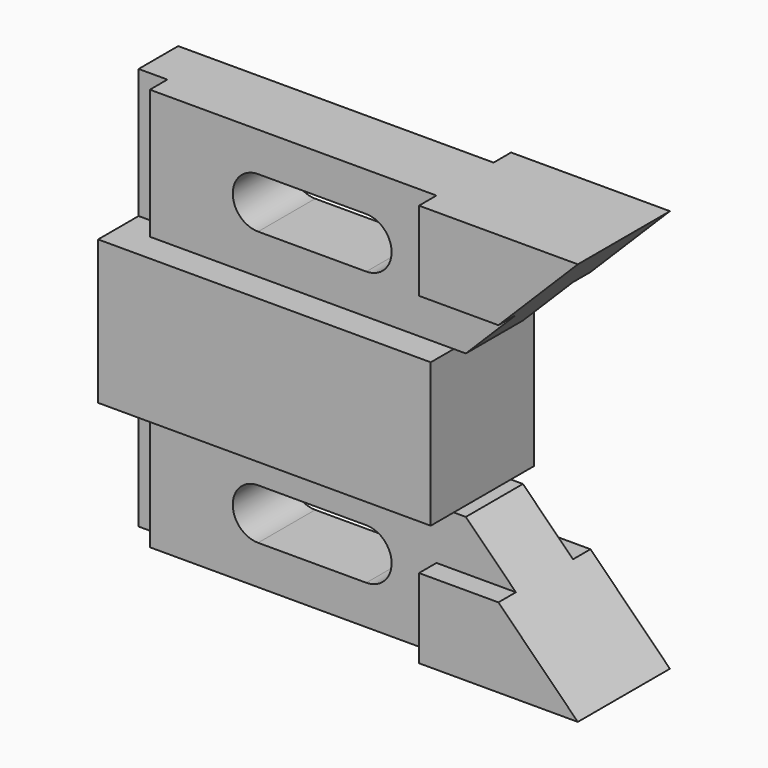
from build123d import *

# Parameters (mm, degrees)
F0_W     = 28.448
F0_H     = 31.75
F1_DEPTH = 73.406
F3_DEPTH = 7.874
F4_W     = 6.35
F4_H     = 28.575
F5_DEPTH = 4.826
F7_DEPTH = 12.7


# Not quite as in the source:
# - a pattern or mirror of a feature is missing from the dataset's text; its kind, count and spacing are read off the source's solid
# - a feature names something its author has since deleted; it is built from what else it names


with BuildPart() as f1:
    # F0 (on Right) → F1 (new body)
    with BuildSketch(Plane.YZ):
        Rectangle(F0_W, F0_H)
    extrude(amount=F1_DEPTH)

    # F2 (on Front) → F3 (join, symmetric)
    with BuildSketch(Plane.XZ):
        Polygon((0, 44.45), (0, 15.875), (73.406, 15.875), (76.073, 15.875), (104.648, 44.45), align=None)
        with BuildLine():
            ThreePointArc((30.226, 24.638), (24.638, 30.226), (30.226, 35.814))
            Line((30.226, 35.814), (54.102, 35.814))
            ThreePointArc((54.102, 35.814), (58.0533126933, 34.1773126933), (59.69, 30.226))
            ThreePointArc((59.69, 30.226), (58.0533126933, 26.2746873067), (54.102, 24.638))
            Line((54.102, 24.638), (30.226, 24.638))
        make_face(mode=Mode.SUBTRACT)
        Polygon((104.648, -44.45), (76.073, -15.875), (73.406, -15.875), (0, -15.875), (0, -44.45), align=None)
        with BuildLine():
            ThreePointArc((54.102, -24.638), (58.0533126933, -26.2746873067), (59.69, -30.226))
            ThreePointArc((59.69, -30.226), (58.0533126933, -34.1773126933), (54.102, -35.814))
            Line((54.102, -35.814), (30.226, -35.814))
            ThreePointArc((30.226, -35.814), (24.638, -30.226), (30.226, -24.638))
            Line((30.226, -24.638), (54.102, -24.638))
        make_face(mode=Mode.SUBTRACT)
    extrude(amount=F3_DEPTH, both=True)

    # F4 (on face) → F5 (cut)
    with BuildSketch(Plane.XZ.offset(7.874)):
        with Locations((3.175, 30.1625)):
            Rectangle(F4_W, F4_H)
    f5 = extrude(amount=-F5_DEPTH, mode=Mode.SUBTRACT)

    # F5_copies: F5 across plane
    add(f5.mirror(Plane(origin=(0, 0, 0), x_dir=(-1, 0, 0), z_dir=(0, 0, -1))), mode=Mode.SUBTRACT)

    # F6 (on Front) → F7 (join, symmetric)
    with BuildSketch(Plane.XZ):
        Polygon((104.648, 44.45), (69.596, 44.45), (69.596, 26.924), (87.122, 26.924), align=None)
    f7 = extrude(amount=F7_DEPTH, both=True)

    # F7_copies: F7 across plane
    add(f7.mirror(Plane(origin=(0, 0, 0), x_dir=(-1, 0, 0), z_dir=(0, 0, -1))))


solid = f1.part
